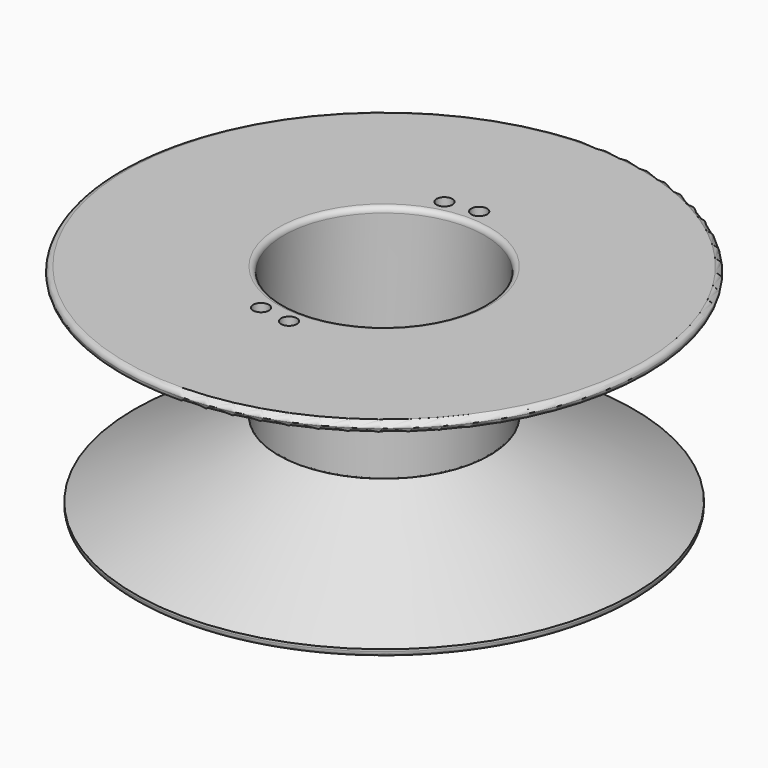
from build123d import *

# Parameters (mm, degrees)
F0_R     = 20
F0_R_2   = 19
F1_DEPTH = 12.5
F2_R     = 50
F2_R_2   = 1.5
F2_R_3   = 20
F3_DEPTH = 2
F6_R     = 0.99999
F7_R     = 1


# Not quite as in the source:
# - a fillet or chamfer is up to 0.001 mm smaller than in the source, because OpenCascade refuses the exact size


with BuildPart() as f1:
    # F0 (on Top) → F1 (new body, symmetric)
    with BuildSketch(Plane.XY):
        Circle(F0_R)
        Circle(F0_R_2, mode=Mode.SUBTRACT)
    extrude(amount=F1_DEPTH, both=True)

    # F2 (on face) → F3 (join)
    with BuildSketch(Plane.XY.offset(12.5)):
        Circle(F2_R)
        with Locations((-5.9464274989, -21.7)):
            Circle(F2_R_2, mode=Mode.SUBTRACT)
        with Locations((0, -22.5)):
            Circle(F2_R_2, mode=Mode.SUBTRACT)
        with Locations((-5.9464274989, 21.7)):
            Circle(F2_R_2, mode=Mode.SUBTRACT)
        Circle(F2_R_3, mode=Mode.SUBTRACT)
        with Locations((0, 22.5)):
            Circle(F2_R_2, mode=Mode.SUBTRACT)
    extrude(amount=-F3_DEPTH)

    # F4 (on Right) → F5 (revolve)
    with BuildSketch(Plane.YZ):
        Polygon((-18.9390927553, -14), (-18.9390927553, -12.5), (-18.9390927553, -12.4), (-20.0090166181, -12.4), (-20.0090166181, -12.5), (-47.3071634769, -26.7197255045), (-47.3071634769, -28.7770535795), align=None)
    revolve(axis=Axis((0, 0, -0.6562490016), (0, 0, -1)))

    # F6 (radius 1 in the source; OpenCascade refuses exactly that, so slightly less here)
    f6_edges = [f1.edges().sort_by_distance(p)[0] for p in [
        (-19, 0, 12.5),
        (-50, 0, 12.5),
        (-50, 0, 10.5),
    ]]
    fillet(f6_edges, radius=F6_R)

    # F7
    f7_edges = [f1.edges().sort_by_distance(p)[0] for p in [
        (0, 47.307163, -28.777054),
        (0, 18.939093, -14),
    ]]
    fillet(f7_edges, radius=F7_R)


solid = f1.part
